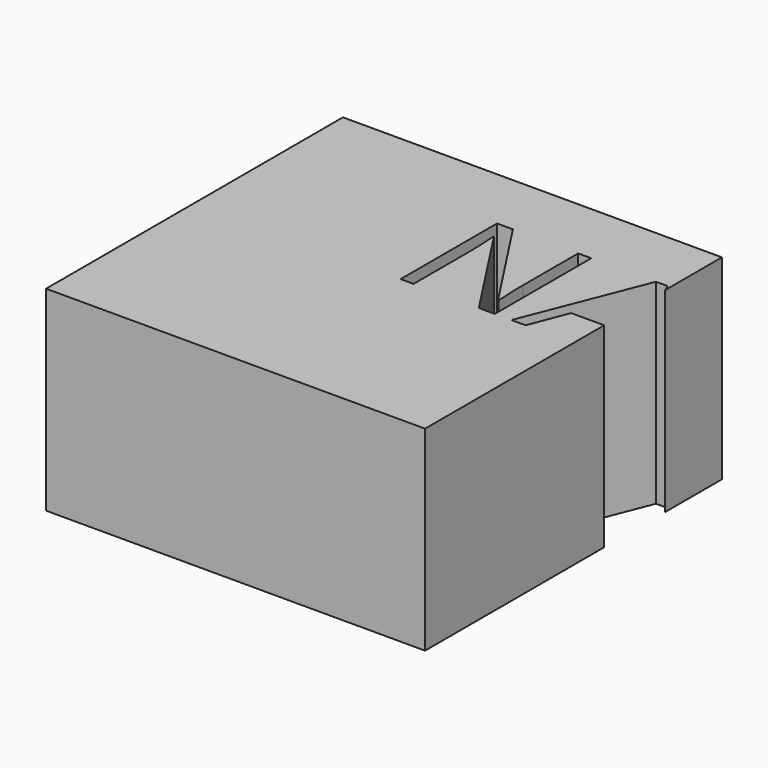
from build123d import *

# Parameters (mm, degrees)
F1_DEPTH = 80


with BuildPart() as f1:
    # F0 (on Top) → F1 (new body)
    with BuildSketch(Plane.XY):
        Polygon((77.5599744916, 46.8204599889), (77.5599744916, 75.9442564845), (-77.5599744916, 75.9442564845), (-77.5599744916, -75.9442564845), (77.5599744916, -75.9442564845), (77.5599744916, 15.7003122036), (64.0222641474, 15.7003122036), (57.9496038182, 0), (52.1362741791, 0), (71.650908618, 49.5753836132), (76.4809427233, 49.5753836132), align=None)
        with BuildLine():
            Line((45.3504544518, 49.3700801502), (45.3504544518, 0))
            Line((45.3504544518, 0), (38.8023545238, 0))
            Line((38.8023545238, 0), (11.8211572957, 41.4280777622))
            Line((11.8211572957, 41.4280777622), (11.5510211601, 41.4280777622))
            add(Edge.make_bspline(
                [(11.5510211601, 41.4280777622), (12.0912934314, 34.1344020999), (12.0912934314, 28.0617417706)],
                knots=[0, 0, 0, 1, 1, 1], degree=2))
            Line((12.0912934314, 28.0617417706), (12.0912934314, 0))
            Line((12.0912934314, 0), (6.7858197274, 0))
            Line((6.7858197274, 0), (6.7858197274, 49.3700801502))
            Line((6.7858197274, 49.3700801502), (13.2690869828, 49.3700801502))
            Line((13.2690869828, 49.3700801502), (40.1854515383, 8.1040840693))
            Line((40.1854515383, 8.1040840693), (40.4555876739, 8.1040840693))
            add(Edge.make_bspline(
                [(40.4555876739, 8.1040840693), (40.3907550014, 9.0117414851), (40.153035202, 13.96063549)],
                knots=[0, 0, 0, 1, 1, 1], degree=2))
            add(Edge.make_bspline(
                [(40.153035202, 13.96063549), (39.9153154026, 18.909529495), (39.9801480752, 21.0382022439)],
                knots=[0, 0, 0, 1, 1, 1], degree=2))
            Line((39.9801480752, 21.0382022439), (39.9801480752, 49.3700801502))
            Line((39.9801480752, 49.3700801502), (45.3504544518, 49.3700801502))
        make_face(mode=Mode.SUBTRACT)
    extrude(amount=F1_DEPTH)


solid = f1.part
